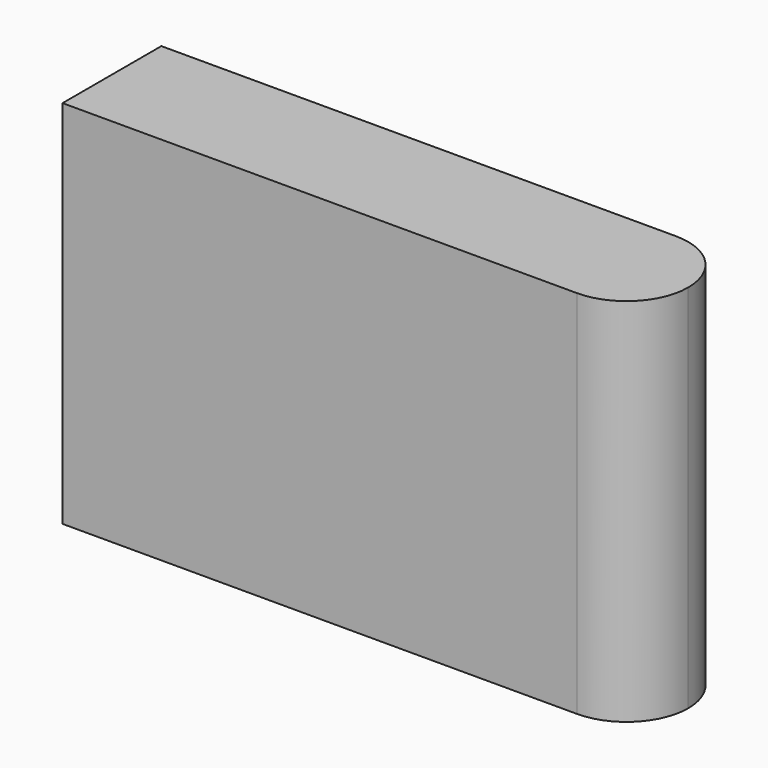
from build123d import *

# Parameters (mm, degrees)
F0_W     = 28
F0_H     = 18
F1_DEPTH = 6
F2_R     = 0.9
F3_DEPTH = 18
F4_R     = 2.99999
F5_SIZE2 = 0.9
F5_SIZE  = 1.5588457268


# Not quite as in the source:
# - a fillet or chamfer is up to 0.001 mm smaller than in the source, because OpenCascade refuses the exact size


with BuildPart() as f1:
    # F0 (on Front) → F1 (new body)
    with BuildSketch(Plane.XZ):
        with Locations((9.4314706177, -13.323269397)):
            Rectangle(F0_W, F0_H)
    extrude(amount=F1_DEPTH)

    # F2 (on face) → F3 (cut)
    with BuildSketch(Plane(origin=(-4.5685293823, 0, 0), x_dir=(0, -1, 0), z_dir=(-1, 0, 0))):
        with Locations((3, -13.323269397)):
            Circle(F2_R)
    extrude(amount=-F3_DEPTH, mode=Mode.SUBTRACT)

    # F4 (radius 3 in the source; OpenCascade refuses exactly that, so slightly less here)
    f4_edges = [f1.edges().sort_by_distance(p)[0] for p in [
        (23.431471, -6, -13.323269),
        (23.431471, 0, -13.323269),
    ]]
    fillet(f4_edges, radius=F4_R)

    # F5
    f5_edges = [f1.edges().sort_by_distance(p)[0] for p in [
        (13.431471, -2.1, -13.323269),
    ]]
    f5_side = f1.faces().sort_by_distance((4.431471, -2.1, -13.323269))[0]
    chamfer(f5_edges, length=F5_SIZE, length2=F5_SIZE2, reference=f5_side)


solid = f1.part
